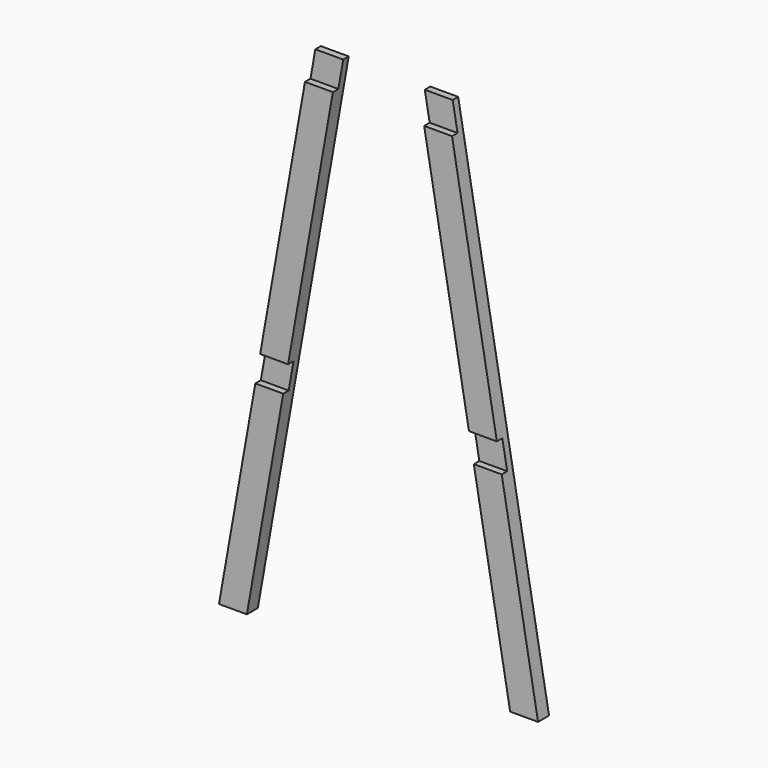
from build123d import *

# Parameters (mm, degrees)
F2_DEPTH = 40
F3_W     = 95.3402874075
F3_H     = 80
F4_DEPTH = 20
F5_DEPTH = 20
F6_W     = 95.3402874075
F6_H     = 80
F7_DEPTH = 20


with BuildPart() as f2:
    # F1 (on Front) → F2 (new body)
    with BuildSketch(Plane.XZ):
        Polygon((-118.7658710491, 1500), (-200, 1500), (-464.4904710627, 0), (-383.2563421118, 0), align=None)
    extrude(amount=F2_DEPTH)

    # F3 (on face) → F4 (cut)
    with BuildSketch(Plane.XZ.offset(40)):
        Polygon((-118.7658710491, 1500), (-200, 1500), (-214.1061584567, 1420), (-132.8720295058, 1420), align=None)
        with Locations((-311.0241389339, 640)):
            Rectangle(F3_W, F3_H)
    extrude(amount=-F4_DEPTH, mode=Mode.SUBTRACT)

    # F3 (on face) → F5 (cut)
    with BuildSketch(Plane.XZ.offset(40)):
        Polygon((-118.7658710491, 1500), (-200, 1500), (-214.1061584567, 1420), (-132.8720295058, 1420), align=None)
        with Locations((-311.0241389339, 640)):
            Rectangle(F3_W, F3_H)
    extrude(amount=-F5_DEPTH, mode=Mode.SUBTRACT)


with BuildPart() as f2b:
    # F1 (on Front) → F2, piece 2 (new body)
    with BuildSketch(Plane.XZ):
        Polygon((118.7658710491, 1500), (383.2563421118, 0), (464.4904710627, 0), (200, 1500), align=None)
    extrude(amount=F2_DEPTH)

    # F6 (on face) → F7 (cut)
    with BuildSketch(Plane.XZ.offset(40)):
        with Locations((166.4360147529, 1460)):
            Rectangle(F6_W, F6_H)
        with Locations((311.0241389339, 640)):
            Rectangle(F6_W, F6_H)
    extrude(amount=-F7_DEPTH, mode=Mode.SUBTRACT)


solid = Compound([f2.part, f2b.part])
